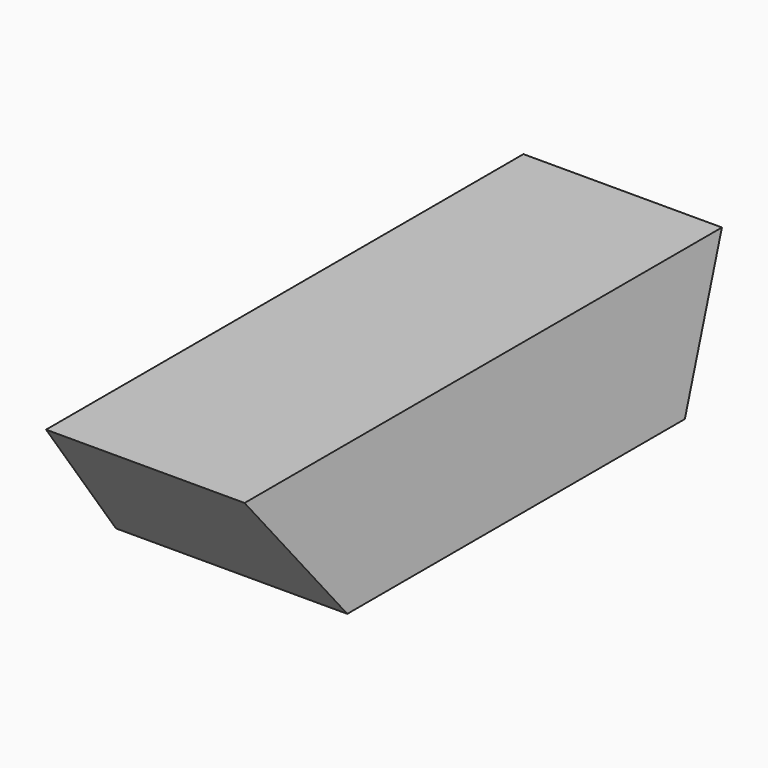
from build123d import *

# Parameters (mm, degrees)
F0_W        = 33.9705549621
F0_H        = 87.9016891122
F1_DEPTH    = 17.9832
F2_T1_DEPTH = 127.9393629633
F3_T1_DEPTH = 181.1359395425


# Not quite as in the source:
# - a fillet or chamfer that OpenCascade refuses, or shapes differently, is made with other operations: its cross-section is extruded or revolved along the edge and cut away or added


with BuildPart() as f1:
    # F0 (on Top) → F1 (new body)
    with BuildSketch(Plane.XY):
        Rectangle(F0_W, F0_H)
    extrude(amount=-F1_DEPTH)

    # F2: chamfer of 12.9794 x 18.1964476933 on 2 edges, made by hand

    # F2_s2 → F2_t1 (cut)
    with BuildSketch(Plane.YZ.offset(-63.9696814817)):
        Polygon((-43.9508445561, 0.2132476933), (-30.9714445561, -17.9832), (-43.9508445561, -17.9832), align=None)
        Polygon((43.9508445561, 0.2132476933), (30.9714445561, -17.9832), (43.9508445561, -17.9832), align=None)
    extrude(amount=F2_T1_DEPTH, mode=Mode.SUBTRACT)

    # F3: chamfer of 4.826 x 18.0108771973 on 1 edges, made by hand

    # F3_s2 → F3_t1 (cut)
    with BuildSketch(Plane.XZ.offset(-90.5679697713)):
        Polygon((12.1592774811, 0), (16.9852774811, -18.0108771973), (16.9852774811, 0), align=None)
    extrude(amount=F3_T1_DEPTH, mode=Mode.SUBTRACT)


solid = f1.part
